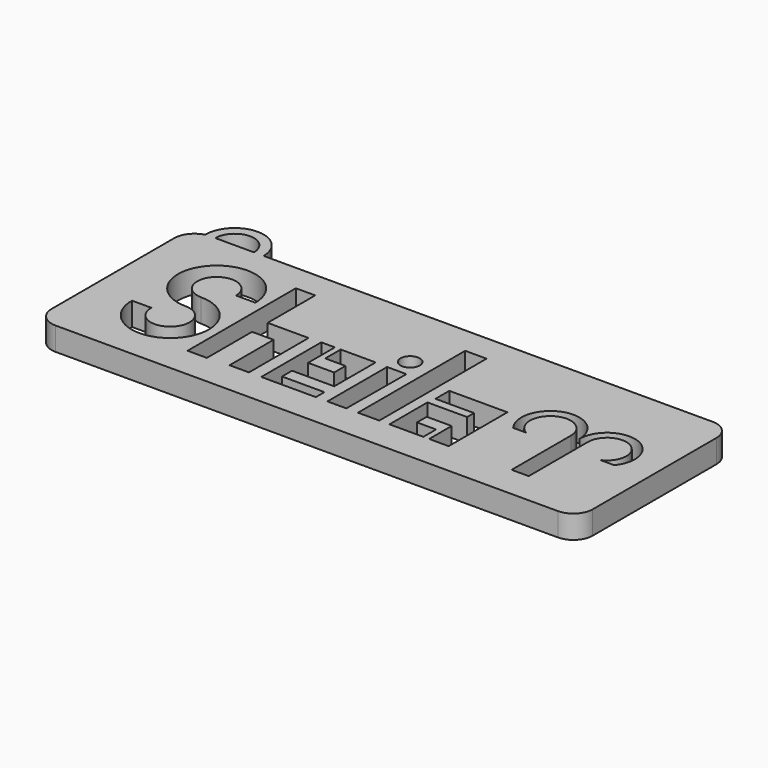
from build123d import *

# Parameters (mm, degrees)
F0_W     = 5.5195543896
F0_H     = 34.641196678
F0_R     = 2.5
F0_W_2   = 1.4996174723
F0_H_2   = 4.8834816366
F0_W_3   = 1.5
F0_H_3   = 4.1201120429
F0_H_4   = 0.1165183634
F1_DEPTH = 6


# Not quite as in the source:
# - a feature names something its author has since deleted; it is built from what else it names


with BuildPart() as f1:
    # F0 (on Top) → F1 (new body)
    with BuildSketch(Plane.XY):
        with BuildLine():
            Line((-67.1787756681, 27.2292699475), (-68.3799158582, 27.2292699475))
            ThreePointArc((-68.3799158582, 27.2292699475), (-69.0335690068, 27.1883203713), (-69.6770007567, 27.0661119853))
            ThreePointArc((-69.6770007567, 27.0661119853), (-72.5165696868, 25.2041102534), (-73.6173242331, 21.9918615726))
            Line((-73.6173242331, 21.9918615726), (-73.6173242331, -17.563536772))
            ThreePointArc((-73.6173242331, -17.563536772), (-72.0921726321, -21.2455784516), (-68.4101309525, -22.7707300525))
            Line((-68.4101309525, -22.7707300525), (61.3826757669, -22.7707300525))
            ThreePointArc((61.3826757669, -22.7707300525), (64.9182096729, -21.3062639585), (66.3826757669, -17.7707300525))
            Line((66.3826757669, -17.7707300525), (66.3826757669, 22.2292699475))
            ThreePointArc((66.3826757669, 22.2292699475), (64.9182096729, 25.7648038534), (61.3826757669, 27.2292699475))
            Line((61.3826757669, 27.2292699475), (-54.6787756681, 27.2292699475))
            Line((-54.6787756681, 27.2292699475), (-57.1787756681, 27.2292699475))
            Line((-57.1787756681, 27.2292699475), (-67.1787756681, 27.2292699475))
        make_face()
        with BuildLine():
            ThreePointArc((-68.3379918337, 19.7292699475), (-67.6057587867, 21.4970369004), (-65.8379918337, 22.2292699475))
            Line((-65.8379918337, 22.2292699475), (58.8826757669, 22.2292699475))
            ThreePointArc((58.8826757669, 22.2292699475), (60.6504427199, 21.4970369004), (61.3826757669, 19.7292699475))
            Line((61.3826757669, 19.7292699475), (61.3826757669, -15.2707300525))
            ThreePointArc((61.3826757669, -15.2707300525), (60.6504427199, -17.0384970055), (58.8826757669, -17.7707300525))
            Line((58.8826757669, -17.7707300525), (-65.8379918337, -17.7707300525))
            ThreePointArc((-65.8379918337, -17.7707300525), (-67.6057587867, -17.0384970055), (-68.3379918337, -15.2707300525))
            Line((-68.3379918337, -15.2707300525), (-68.3379918337, 19.7292699475))
        make_face(mode=Mode.SUBTRACT)
        with BuildLine():
            Line((58.8826757669, 22.2292699475), (-65.8379918337, 22.2292699475))
            ThreePointArc((-65.8379918337, 22.2292699475), (-67.6057587867, 21.4970369004), (-68.3379918337, 19.7292699475))
            Line((-68.3379918337, 19.7292699475), (-68.3379918337, -15.2707300525))
            ThreePointArc((-68.3379918337, -15.2707300525), (-67.6057587867, -17.0384970055), (-65.8379918337, -17.7707300525))
            Line((-65.8379918337, -17.7707300525), (58.8826757669, -17.7707300525))
            ThreePointArc((58.8826757669, -17.7707300525), (60.6504427199, -17.0384970055), (61.3826757669, -15.2707300525))
            Line((61.3826757669, -15.2707300525), (61.3826757669, 19.7292699475))
            ThreePointArc((61.3826757669, 19.7292699475), (60.6504427199, 21.4970369004), (58.8826757669, 22.2292699475))
        make_face()
        with BuildLine():
            ThreePointArc((-53.204651922, 0.2162606642), (-60.2757197339, 17.287328476), (-43.204651922, 10.2162606642))
            Line((-43.204651922, 10.2162606642), (-48.204651922, 10.2162606642))
            ThreePointArc((-48.204651922, 10.2162606642), (-56.7401858279, 13.7517945701), (-53.204651922, 5.2162606642))
            ThreePointArc((-53.204651922, 5.2162606642), (-46.1867208519, -11.9075475516), (-63.203530925, -4.6340106369))
            Line((-63.203530925, -4.6340106369), (-58.2024095508, -4.6340106369))
            ThreePointArc((-58.2024095508, -4.6340106369), (-49.7224574627, -8.371819846), (-53.204651922, 0.2162606642))
        make_face(mode=Mode.SUBTRACT)
        Polygon((-7.8910876493, -14.387637473), (-21.9972077757, -14.387637473), (-21.9972077757, 4.8834816366), (-21.9972077757, 5), (-18.4776540846, 5), (-16.9780366123, 5), (-7.9369102418, 5), (-7.9369102418, 4.8834816366), (-7.9369102418, -8.3816020689), (-18.8480350176, -8.3816020689), (-18.8480350176, -11.6097754424), (-7.8910876493, -11.6097754424), align=None, mode=Mode.SUBTRACT)
        Polygon((-40.7681576908, -14.7364697516), (-40.7681576908, 20.253559205), (-35.7681576908, 20.253559205), (-35.7681576908, 4.8834816366), (-25.1815660298, 4.8834816366), (-25.1776284749, 4.8834816366), (-25.1776284749, -14.387637473), (-30.1955331862, -14.387637473), (-30.1955331862, -0.1466480026), (-35.7681576908, -0.1466480026), (-35.7681576908, -14.7364697516), align=None, mode=Mode.SUBTRACT)
        Polygon((0, -14.387637473), (-4.8910876493, -14.387637473), (-4.8910876493, 4.8834816366), (0.1088994695, 4.8721321267), align=None, mode=Mode.SUBTRACT)
        Polygon((19.8960285634, -14.387637473), (11.1452508718, -14.387637473), (11.1452508718, -2.1165183634), (21.3960285634, -2.1165183634), (21.3960285634, 0.1236622645), (11.4239600822, 0.1236622645), (11.4239600822, 4.5901425229), (26.3825752896, 4.5901425229), (26.4385476336, 4.5901425229), (26.4385476336, -14.387637473), (21.3960285634, -14.387637473), align=None, mode=Mode.SUBTRACT)
        with Locations((5.7597771948, 2.932960866)):
            Rectangle(F0_W, F0_H, mode=Mode.SUBTRACT)
        with BuildLine():
            Line((47.2346405685, -14.5181566477), (42.8212322295, -14.5181566477))
            Line((42.8212322295, -14.5181566477), (42.8212322295, 4.6019549295))
            ThreePointArc((42.8212322295, 4.6019549295), (34.8761091537, 9.1588015867), (34.9547580095, 0))
            Line((34.9547580095, 0), (31.6197408739, 0))
            ThreePointArc((31.6197408739, 0), (35.1094377398, 11.6965380784), (45.0419035554, 4.6019549295))
            ThreePointArc((45.0419035554, 4.6019549295), (54.6550720871, 11.3354460366), (57.6981913518, 0))
            Line((57.6981913518, 0), (54.089111107, 0))
            ThreePointArc((54.089111107, 0), (54.9781676596, 8.7299615773), (47.2346405685, 4.6019549295))
            Line((47.2346405685, 4.6019549295), (47.2346405685, -14.5181566477))
        make_face(mode=Mode.SUBTRACT)
        with Locations((-2.6396652684, 9.5321238041)):
            Circle(F0_R, mode=Mode.SUBTRACT)
        with BuildLine():
            Line((-68.6173242331, 27.2292699475), (-68.3799158582, 27.2292699475))
            Line((-68.3799158582, 27.2292699475), (-67.1787756681, 27.2292699475))
            ThreePointArc((-67.1787756681, 27.2292699475), (-62.1787756681, 32.2292699475), (-57.1787756681, 27.2292699475))
            Line((-57.1787756681, 27.2292699475), (-54.6787756681, 27.2292699475))
            ThreePointArc((-54.6787756681, 27.2292699475), (-62.2356669727, 34.7290541697), (-69.6779125693, 27.1154906119))
            ThreePointArc((-69.6779125693, 27.1154906119), (-69.1506612176, 27.2007437391), (-68.6173242331, 27.2292699475))
        make_face()
        Polygon((-16.9780366123, 0), (-18.4776540846, 0), (-18.4776540846, -3.6654266296), (-11.7318434641, -3.6654266296), (-11.7318434641, 0), align=None)
        Polygon((14.9498761296, -10.2675254301), (19.8960285634, -10.2675254301), (21.3960285634, -10.2675254301), (21.3960285634, -7.1165183634), (14.9498761296, -7.1165183634), align=None)
        with Locations((-17.7278453484, 2.4417408183)):
            Rectangle(F0_W_2, F0_H_2)
        with Locations((20.6460285634, -12.3275814516)):
            Rectangle(F0_W_3, F0_H_3)
        with Locations((-17.7278453484, 4.9417408183)):
            Rectangle(F0_W_2, F0_H_4)
        with BuildLine():
            ThreePointArc((-69.6770007567, 27.0661119853), (-69.0335690068, 27.1883203713), (-68.3799158582, 27.2292699475))
            Line((-68.3799158582, 27.2292699475), (-68.6173242331, 27.2292699475))
            ThreePointArc((-68.6173242331, 27.2292699475), (-69.1506612176, 27.2007437391), (-69.6779125693, 27.1154906119))
            ThreePointArc((-69.6779125693, 27.1154906119), (-69.6774973076, 27.0908005481), (-69.6770007567, 27.0661119853))
        make_face()
    extrude(amount=F1_DEPTH)


solid = f1.part
